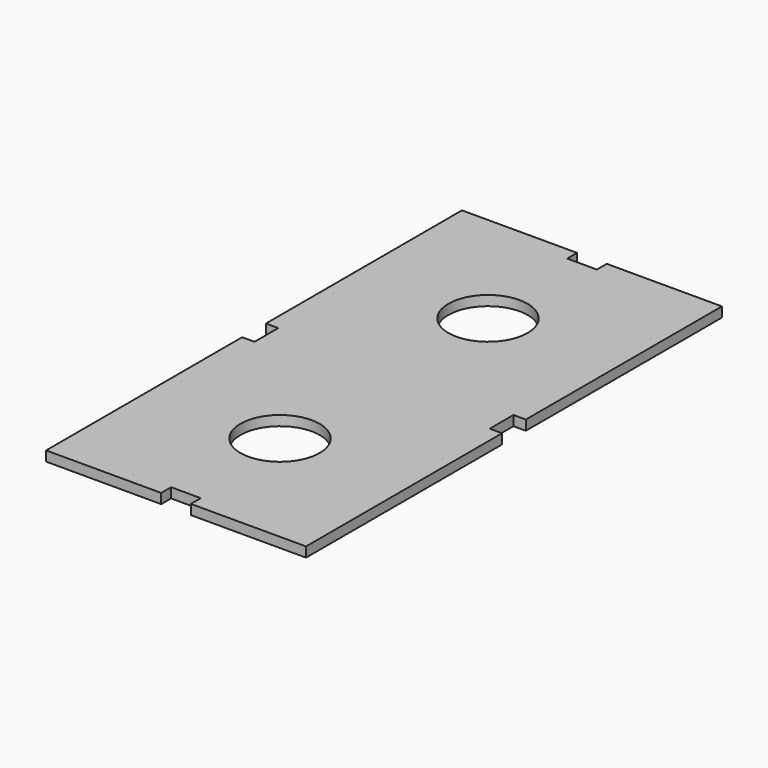
from build123d import *

# Parameters (mm, degrees)
F1_DEPTH = 12.7


with BuildPart() as f1:
    # F0 (on Top) → F1 (new body)
    with BuildSketch(Plane.XY):
        with BuildLine():
            Line((166.6875, -333.375), (166.6875, -166.6875))
            Line((166.6875, -166.6875), (50.8, -166.6875))
            ThreePointArc((50.8, -166.6875), (0, -217.4875), (-50.8, -166.6875))
            Line((-50.8, -166.6875), (-166.6875, -166.6875))
            Line((-166.6875, -166.6875), (-166.6875, -333.375))
            Line((-166.6875, -333.375), (-19.05, -333.375))
            Line((-19.05, -333.375), (-19.05, -317.5))
            Line((-19.05, -317.5), (19.05, -317.5))
            Line((19.05, -317.5), (19.05, -333.375))
            Line((19.05, -333.375), (166.6875, -333.375))
        make_face()
        with BuildLine():
            Line((50.8, 166.6875), (166.6875, 166.6875))
            Line((166.6875, 166.6875), (166.6875, 333.375))
            Line((166.6875, 333.375), (19.05, 333.375))
            Line((19.05, 333.375), (19.05, 317.5))
            Line((19.05, 317.5), (-19.05, 317.5))
            Line((-19.05, 317.5), (-19.05, 333.375))
            Line((-19.05, 333.375), (-166.6875, 333.375))
            Line((-166.6875, 333.375), (-166.6875, 166.6875))
            Line((-166.6875, 166.6875), (-50.8, 166.6875))
            ThreePointArc((-50.8, 166.6875), (0, 217.4875), (50.8, 166.6875))
        make_face()
        with BuildLine():
            Line((50.8, -166.6875), (166.6875, -166.6875))
            Line((166.6875, -166.6875), (166.6875, -19.05))
            Line((166.6875, -19.05), (150.8125, -19.05))
            Line((150.8125, -19.05), (150.8125, 19.05))
            Line((150.8125, 19.05), (166.6875, 19.05))
            Line((166.6875, 19.05), (166.6875, 166.6875))
            Line((166.6875, 166.6875), (50.8, 166.6875))
            ThreePointArc((50.8, 166.6875), (0, 115.8875), (-50.8, 166.6875))
            Line((-50.8, 166.6875), (-166.6875, 166.6875))
            Line((-166.6875, 166.6875), (-166.6875, 19.05))
            Line((-166.6875, 19.05), (-150.8125, 19.05))
            Line((-150.8125, 19.05), (-150.8125, -19.05))
            Line((-150.8125, -19.05), (-166.6875, -19.05))
            Line((-166.6875, -19.05), (-166.6875, -166.6875))
            Line((-166.6875, -166.6875), (-50.8, -166.6875))
            ThreePointArc((-50.8, -166.6875), (0, -115.8875), (50.8, -166.6875))
        make_face()
    extrude(amount=F1_DEPTH)


solid = f1.part
